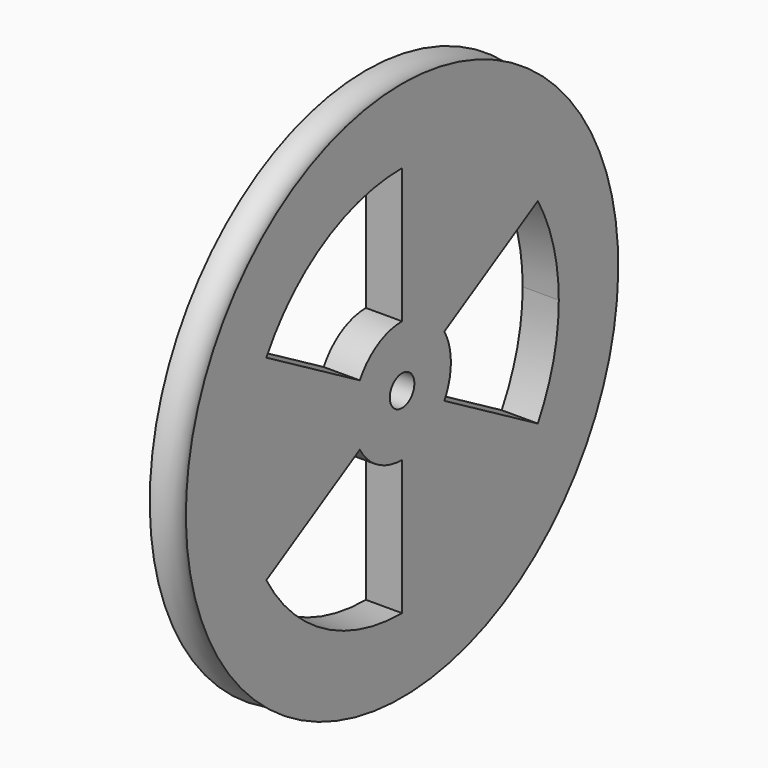
from build123d import *

# Parameters (mm, degrees)
F3_DEPTH      = 82
F3_DEPTH_BACK = 25.4
F4_R          = 1.6002
F5_DEPTH      = 3.7619021022


# Not quite as in the source:
# - an extrude ends at something that could not be found from the text; its depth is read off the source's solid


with BuildPart() as f1:
    # F0 (on Front) → F1 (revolve)
    with BuildSketch(Plane.XZ):
        with BuildLine():
            Line((0, 28.125), (0, 0))
            Line((0, 0), (3.7609021022, 0))
            Line((3.7609021022, 0), (3.7609021022, 28.125))
            ThreePointArc((3.7609021022, 28.125), (1.8804510511, 27.2531215698), (0, 28.125))
        make_face()
    revolve(axis=Axis((1.8804510511, 0, 0), (1, 0, 0)))

    # F2 (on Right) → F3 (cut, two sides)
    with BuildSketch(Plane.YZ) as f3_sk:
        with BuildLine():
            ThreePointArc((-5.499261314, 3.175), (-3.175, 5.499261314), (0, 6.35))
            Line((0, 6.35), (0, 20.391961195))
            ThreePointArc((0, 20.391961195), (-10.1959805975, 17.6599564279), (-17.6599564279, 10.1959805975))
            Line((-17.6599564279, 10.1959805975), (-5.499261314, 3.175))
        make_face()
        with BuildLine():
            Line((0, -20.391961195), (0, -6.35))
            ThreePointArc((0, -6.35), (-3.175, -5.499261314), (-5.499261314, -3.175))
            Line((-5.499261314, -3.175), (-17.6599564279, -10.1959805975))
            ThreePointArc((-17.6599564279, -10.1959805975), (-10.1959805975, -17.6599564279), (0, -20.391961195))
        make_face()
        with BuildLine():
            ThreePointArc((5.499261314, 3.175), (6.1336289969, 1.6435009364), (6.35, 0))
            ThreePointArc((6.35, 0), (6.1336289969, -1.6435009364), (5.499261314, -3.175))
            Line((5.499261314, -3.175), (17.6599564279, -10.1959805975))
            ThreePointArc((17.6599564279, -10.1959805975), (19.6971219669, -5.2778279243), (20.391961195, 0))
            ThreePointArc((20.391961195, 0), (19.6971219669, 5.2778279243), (17.6599564279, 10.1959805975))
            Line((17.6599564279, 10.1959805975), (5.499261314, 3.175))
        make_face()
    extrude(amount=-F3_DEPTH, mode=Mode.SUBTRACT)
    extrude(f3_sk.sketch, amount=F3_DEPTH_BACK, mode=Mode.SUBTRACT)

    # F4 (on face) → F5 (cut, through all)
    with BuildSketch(Plane(origin=(0, 0, 0), x_dir=(0, -1, 0), z_dir=(-1, 0, 0))):
        Circle(F4_R)
    extrude(amount=-F5_DEPTH, mode=Mode.SUBTRACT)


solid = f1.part
